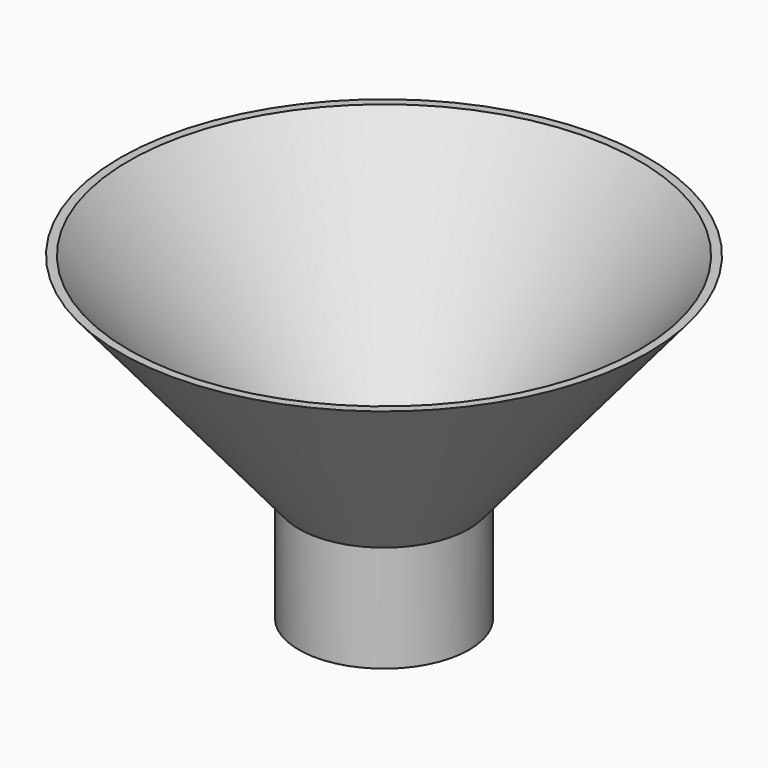
from build123d import *

# Parameters (mm, degrees)
F0_R                   = 20
F0_R_2                 = 18
F1_DEPTH               = 25
F2_R                   = 20
F2_R_2                 = 18
F3_DEPTH               = 50
DRAFT_F3_DRAFTED_ANGLE = -40
F4_DEPTH               = 50
F4_TAPER               = -40


# Not quite as in the source:
# - an extrude with a draft is written as a straight extrude whose walls are then drafted


with BuildPart() as f1:
    # F0 (on Top) → F1 (new body)
    with BuildSketch(Plane.XY):
        Circle(F0_R)
        Circle(F0_R_2, mode=Mode.SUBTRACT)
    extrude(amount=F1_DEPTH)


with BuildPart() as f3_drafted:
    # F2 (on face) → F3 (new body)
    with BuildSketch(Plane.XY.offset(25)):
        Circle(F2_R)
        Circle(F2_R_2, mode=Mode.SUBTRACT)
    extrude(amount=F3_DEPTH)

    # draft_F3_drafted
    draft_f3_drafted_walls = [f3_drafted.faces().sort_by_distance(p)[0] for p in [
        (-20, 0, 58.3333333333),
        (-18, 0, 58.3333333333),
    ]]
    draft(draft_f3_drafted_walls, neutral_plane=Plane.XY.offset(25), angle=DRAFT_F3_DRAFTED_ANGLE)


with BuildPart() as f1_1:
    add(f1.part)

    # join_F3_drafted: union F3_drafted
    add(f3_drafted.part)

    # F2 (on face) → F4 (cut)
    with BuildSketch(Plane.XY.offset(25)):
        Circle(F2_R_2)
    extrude(amount=F4_DEPTH, taper=F4_TAPER, mode=Mode.SUBTRACT)


solid = f1_1.part
